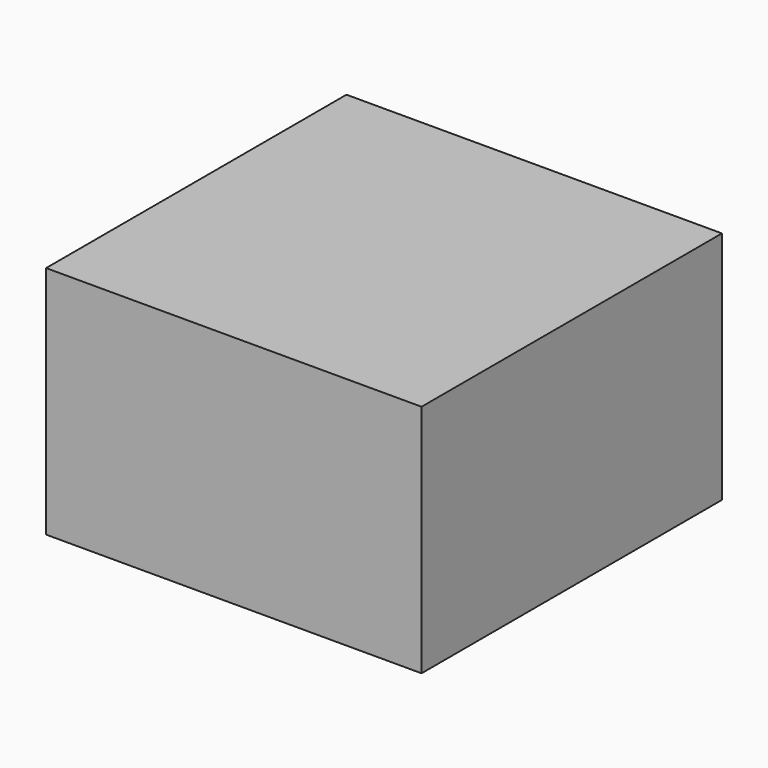
from build123d import *

# Parameters (mm, degrees)
F0_W     = 50.8
F0_H     = 50.8
F1_DEPTH = 25.4
F2_DEPTH = 6.35
F3_DEPTH = 20.828


# Not quite as in the source:
# - a feature names something its author has since deleted; it is built from what else it names


with BuildPart() as f1:
    # F0 (on Top) → F1 (new body)
    with BuildSketch(Plane.XY):
        with Locations((-25.4, 25.4)):
            Rectangle(F0_W, F0_H)
    extrude(amount=F1_DEPTH)

    # F2 (add): a face of the model
    f2_faces = [f1.faces().sort_by_distance(p)[0] for p in [
        (-25.4, 25.4, 25.4),
    ]]
    extrude(f2_faces, amount=F2_DEPTH)

    # F0 (on Top) → F3 (join)
    with BuildSketch(Plane.XY):
        with Locations((-25.4, 25.4)):
            Rectangle(F0_W, F0_H)
    extrude(amount=F3_DEPTH)


solid = f1.part
